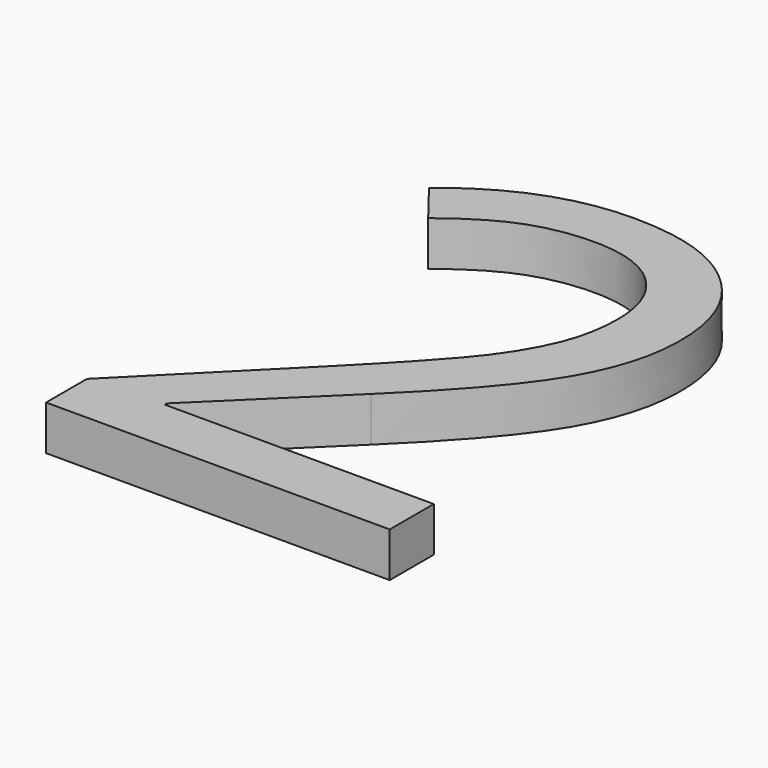
from build123d import *

# Parameters (mm, degrees)
F0_TEXT_SIZE = 416.6666666667
F1_DEPTH     = 25.4


# Not quite as in the source:
# - Text() gives the source's letters only with a copy of the font that has no kerning and outlines rounded to 1/6400 em; it was checked with that copy


with BuildPart() as f1:
    # F0 (on Top) → F1 (new body)
    with BuildSketch(Plane.XY):
        with Locations((0, 0)):
            Text('2', F0_TEXT_SIZE, font='Open Sans', text_align=(TextAlign.LEFT, TextAlign.BOTTOM))
    extrude(amount=F1_DEPTH)


solid = f1.part
